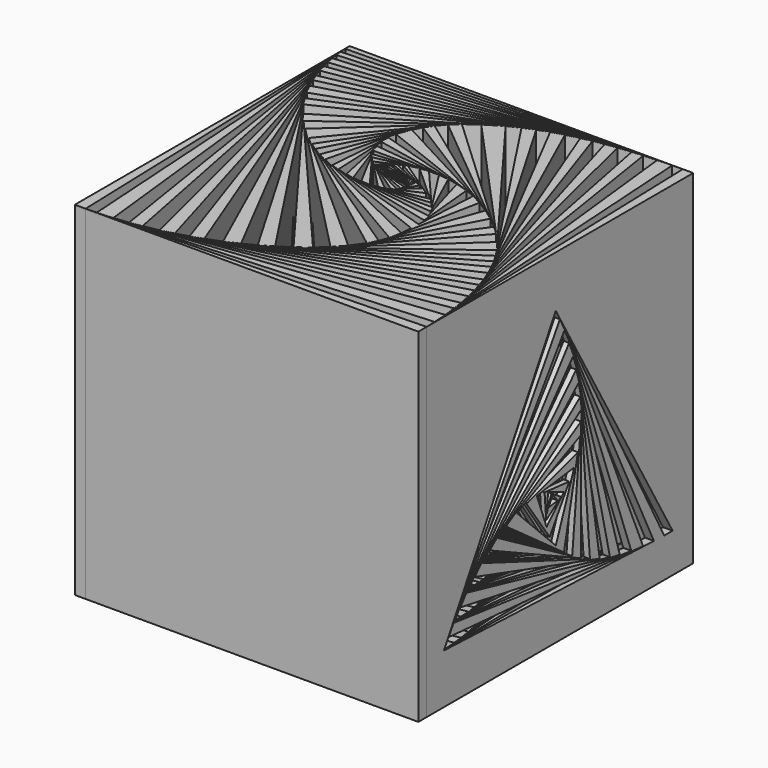
from build123d import *

# Parameters (mm, degrees)
F1_DEPTH = 254
F3_DEPTH = 254.001


with BuildPart() as f1:
    # F0 (on Top) → F1 (new body)
    with BuildSketch(Plane.XY):
        Polygon((-126.8681881938, 122.7877680736), (-127, 127), (-127, -127), (-119.0516725183, -127), align=None)
        Polygon((119.2926133431, 127), (-127, 127), (-126.8681881938, 122.7877680736), (111.5874118838, 126.8681508372), align=None)
    extrude(amount=F1_DEPTH)


with BuildPart() as f1b:
    # F0 (on Top) → F1, piece 2 (new body)
    with BuildSketch(Plane.XY):
        Polygon((-126.0531846551, 113.5256776399), (-126.5785198377, 118.234531984), (-110.9932006372, -126.7478292381), (-99.3302639061, -126.005855037), align=None)
        Polygon((100.7129844798, 126.4739481031), (-126.5785198377, 118.234531984), (-126.0531846551, 113.5256776399), (90.920474554, 125.9147991458), align=None)
    extrude(amount=F1_DEPTH)


with BuildPart() as f1c:
    # F0 (on Top) → F1, piece 3 (new body)
    with BuildSketch(Plane.XY):
        Polygon((-125.3309426111, 108.9235324963), (-88.6490839555, -124.8142276878), (-79.7889641882, -123.4237563291), (-124.2173594964, 103.2422242495), align=None)
        Polygon((82.861461887, 125.281587882), (-125.3309426111, 108.9235324963), (-124.2173594964, 103.2422242495), (73.0560890227, 124.2380037209), align=None)
    extrude(amount=F1_DEPTH)


with BuildPart() as f1d:
    # F0 (on Top) → F1, piece 4 (new body)
    with BuildSketch(Plane.XY):
        Polygon((-122.9498802149, 98.0990388663), (-68.8848311302, -121.2864566216), (-59.508664245, -118.9758074069), (-121.2575487035, 92.3084404823), align=None)
        Polygon((64.6451510187, 123.1163378158), (-122.9498802149, 98.0990388663), (-121.2575487035, 92.3084404823), (56.6793703964, 121.7962442832), align=None)
    extrude(amount=F1_DEPTH)


with BuildPart() as f1e:
    # F0 (on Top) → F1, piece 5 (new body)
    with BuildSketch(Plane.XY):
        Polygon((-119.2080548208, 86.2513609913), (-50.643371318, -116.3848809459), (-42.072519088, -113.4848184256), (-116.9805984588, 80.4835443898), align=None)
        Polygon((48.9444702898, 120.2331074005), (-119.2080548208, 86.2513609913), (-116.9805984588, 80.4835443898), (39.418420978, 117.9510152476), align=None)
    extrude(amount=F1_DEPTH)


with BuildPart() as f1f:
    # F0 (on Top) → F1, piece 6 (new body)
    with BuildSketch(Plane.XY):
        Polygon((-114.0299334632, 73.9299803487), (-31.4888725769, -109.3975506806), (-21.7236330528, -105.0008666387), (-110.0116567717, 66.1407650009), align=None)
        Polygon((30.5370410153, 115.4031382194), (-114.0299334632, 73.9299803487), (-110.0116567717, 66.1407650009), (22.4576933662, 112.5713237272), align=None)
    extrude(amount=F1_DEPTH)


with BuildPart() as f1g:
    # F0 (on Top) → F1, piece 7 (new body)
    with BuildSketch(Plane.XY):
        Polygon((-106.4882692452, 60.0895785941), (-12.9864915382, -100.4935766831), (-4.2246983161, -95.3919006028), (-102.1543719548, 53.5003234443), align=None)
        Polygon((14.2621881215, 109.2357061648), (-106.4882692452, 60.0895785941), (-102.1543719548, 53.5003234443), (5.7810312128, 105.1752827516), align=None)
    extrude(amount=F1_DEPTH)


with BuildPart() as f1h:
    # F0 (on Top) → F1, piece 8 (new body)
    with BuildSketch(Plane.XY):
        Polygon((-95.2082875467, 44.2061987353), (4.7235736363, -89.5064263442), (13.7388739494, -82.7687249575), (-89.3516796687, 37.3804831481), align=None)
        Polygon((-6.3725892117, 97.8379215944), (-95.2082875467, 44.2061987353), (-89.3516796687, 37.3804831481), (-15.4159002419, 91.2490879865), align=None)
    extrude(amount=F1_DEPTH)


with BuildPart() as f1i:
    # F0 (on Top) → F1, piece 9 (new body)
    with BuildSketch(Plane.XY):
        Polygon((-82.4406216858, 30.2987939235), (21.2429796219, -75.9447137933), (28.1362773895, -68.2066711256), (-73.7012457184, 22.5134761845), align=None)
        Polygon((-21.4167941901, 85.7920529864), (-82.4406216858, 30.2987939235), (-73.7012457184, 22.5134761845), (-26.4319034603, 79.7223904415), align=None)
    extrude(amount=F1_DEPTH)


with BuildPart() as f1j:
    # F0 (on Top) → F1, piece 10 (new body)
    with BuildSketch(Plane.XY):
        Polygon((-67.6123478435, 17.92552461), (34.6745146372, -59.1470723376), (38.187583362, -52.5778597304), (-62.191322811, 14.3130401118), align=None)
        Polygon((-30.3811760363, 73.7959690255), (-67.6123478435, 17.92552461), (-62.191322811, 14.3130401118), (-33.6265531217, 67.7273225702), align=None)
    extrude(amount=F1_DEPTH)


with BuildPart() as f1k:
    # F0 (on Top) → F1, piece 11 (new body)
    with BuildSketch(Plane.XY):
        Polygon((-55.9045816766, 10.6394204058), (40.63624374, -45.7736354381), (42.3923361661, -36.9523441909), (-49.5893935967, 7.5818378175), align=None)
        Polygon((-37.5137914336, 57.7661951799), (-55.9045816766, 10.6394204058), (-49.5893935967, 7.5818378175), align=None)
    extrude(amount=F1_DEPTH)


with BuildPart() as f1l:
    # F0 (on Top) → F1, piece 12 (new body)
    with BuildSketch(Plane.XY):
        Polygon((-41.9461483319, 4.5991316782), (42.8538182602, -28.4932750414), (43.2045911016, -22.0635310509), (-35.8799262071, 2.699657456), align=None)
        Polygon((42.3923361661, -36.9523441909), (53.9119721681, 20.913667144), (45.7862644887, 25.2591147985), (43.2045911016, -22.0635310509), (42.8538182602, -28.4932750414), align=None)
        Polygon((29.1134557679, 30.991217705), (-38.0250574646, 51.6334504213), (-37.7312351463, 44.9309046261), (21.4549733149, 32.5883056147), align=None)
        Polygon((-37.7312351463, 44.9309046261), (-38.0250574646, 51.6334504213), (-41.9461483319, 4.5991316782), (-35.8799262071, 2.699657456), align=None)
    extrude(amount=F1_DEPTH)


with BuildPart() as f1m:
    # F0 (on Top) → F1, piece 13 (new body)
    with BuildSketch(Plane.XY):
        Polygon((-28.5686212395, 0.9403759842), (42.6506705396, -16.196753573), (40.9614547645, -10.3084917096), (-22.7560883308, 0), align=None)
        Polygon((42.6506705396, -16.196753573), (38.4668684028, 28.1154417754), (29.1134557679, 30.991217705), (40.9614547645, -10.3084917096), align=None)
        Polygon((13.8678958486, 33.4607075332), (-36.5496441153, 39.2579804339), (-34.5127332434, 33.4607075332), (6.4919767901, 33.4607075332), align=None)
        Polygon((-36.5496441153, 39.2579804339), (-28.5686212395, 0.9403759842), (-22.7560883308, 0), (-34.5127332434, 33.4607075332), align=None)
    extrude(amount=F1_DEPTH)


with BuildPart() as f1n:
    # F0 (on Top) → F1, piece 14 (new body)
    with BuildSketch(Plane.XY):
        Polygon((-16.3723659513, -0.53218918), (38.5998311843, -5.1150339177), (35.6616473557, -0.53218918), (-10.06167382, -0.53218918), align=None)
        Polygon((38.5998311843, -5.1150339177), (21.4549733149, 32.5883056147), (13.8678958486, 33.4607075332), (35.6616473557, -0.53218918), align=None)
        Polygon((0, 32.847757844), (-32.5457947044, 29.7748980058), (-30.1643975353, 26.5649343163), (-7.5473354002, 31.2757530868), align=None)
        Polygon((-32.5457947044, 29.7748980058), (-16.3723659513, -0.53218918), (-10.06167382, -0.53218918), (-30.1643975353, 26.5649343163), align=None)
    extrude(amount=F1_DEPTH)


with BuildPart() as f1o:
    # F0 (on Top) → F1, piece 15 (new body)
    with BuildSketch(Plane.XY):
        Polygon((-4.4250614438, 0), (32.2347954518, 3.4612951674), (28.5073621781, 6.8593647764), (0, 0.9216786153), align=None)
        Polygon((32.2347954518, 3.4612951674), (6.4919767901, 33.4607075332), (0, 32.847757844), (28.5073621781, 6.8593647764), align=None)
        Polygon((-10.146825692, 30.0936856058), (-26.41552278, 22.6958130896), (-23.6386533221, 20.4068586177), (-12.6147075733, 28.3218022504), align=None)
        Polygon((-26.41552278, 22.6958130896), (-4.4250614438, 0), (0, 0.9216786153), (-23.6386533221, 20.4068586177), align=None)
    extrude(amount=F1_DEPTH)


with BuildPart() as f1p:
    # F0 (on Top) → F1, piece 16 (new body)
    with BuildSketch(Plane.XY):
        Polygon((3.329507322, 2.4357070944), (22.300748578, 11.0625088306), (17.0034638905, 14.1694764109), (5.6537325265, 4.4301497601), align=None)
        Polygon((22.300748578, 11.0625088306), (-7.5473354002, 31.2757530868), (-10.146825692, 30.0936856058), (17.0034638905, 14.1694764109), align=None)
        Polygon((-14.1419558573, 26.6465228342), (-21.2695208096, 18.8281065506), (-19.3345417112, 17.7933227858), (-15.1082700185, 24.9989867473), align=None)
        Polygon((-21.2695208096, 18.8281065506), (3.329507322, 2.4357070944), (5.6537325265, 4.4301497601), (-19.3345417112, 17.7933227858), align=None)
    extrude(amount=F1_DEPTH)


with BuildPart() as f1q:
    # F0 (on Top) → F1, piece 17 (new body)
    with BuildSketch(Plane.XY):
        Polygon((7.0708972275, 6.5567984207), (13.3175243975, 15.9307133189), (9.3487022791, 17.4795096335), (7.6296184466, 9.2360226677), align=None)
        Polygon((13.3175243975, 15.9307133189), (-12.6147075733, 28.3218022504), (-14.1419558573, 26.6465228342), (9.3487022791, 17.4795096335), align=None)
        Polygon((-15.6042921852, 22.9375944176), (-17.0736371197, 16.8312213949), (-14.9665841049, 16.1833923534), (-15.3697161374, 20.4531127634), align=None)
        Polygon((-17.0736371197, 16.8312213949), (7.0708972275, 6.5567984207), (7.6296184466, 9.2360226677), (-14.9665841049, 16.1833923534), align=None)
    extrude(amount=F1_DEPTH)


with BuildPart() as f1r:
    # F0 (on Top) → F1, piece 18 (new body)
    with BuildSketch(Plane.XY):
        Polygon((7.4143406474, 11.5161094355), (6.7766325671, 18.2703114997), (4.0880434359, 18.8309856571), (6.4859856679, 13.5576593431), align=None)
        Polygon((6.7766325671, 18.2703114997), (-15.1082700185, 24.9989867473), (-15.6042921852, 22.9375944176), (4.0880434359, 18.8309856571), align=None)
        Polygon((-13.2669719556, 15.8289579035), (7.4143406474, 11.5161094355), (6.4859856679, 13.5576593431), (-10.9204565094, 15.5591432633), align=None)
    extrude(amount=F1_DEPTH)


with BuildPart() as f1s:
    # F0 (on Top) → F1, piece 19 (new body)
    with BuildSketch(Plane.XY):
        Polygon((5.5390247102, 14.6612009808), (1.7969907997, 19.0219829078), (0.2486957437, 19.0219829078), (4.4496764816, 15.5591432633), align=None)
        Polygon((1.7969907997, 19.0219829078), (-15.3697161374, 20.4531127634), (-14.7189377641, 19.0219829078), (0.2486957437, 19.0219829078), align=None)
        Polygon((-12.6174739078, 17.1062087167), (-10.9204565094, 15.5591432633), (-10.064965114, 15.5591432633), (-11.738615487, 16.5735361145), align=None)
        Polygon((-10.064965114, 15.5591432633), (-10.9204565094, 15.5591432633), (5.5390247102, 14.6612009808), (4.4496764816, 15.5591432633), align=None)
    extrude(amount=F1_DEPTH)


with BuildPart() as f1t:
    # F0 (on Top) → F1, piece 20 (new body)
    with BuildSketch(Plane.XY):
        Polygon((3.1098938176, 16.3492539877), (-1.1916278715, 18.8859926014), (-2.9219602182, 18.6164617837), (1.7273046558, 16.8689311728), align=None)
        Polygon((-1.1916278715, 18.8859926014), (-13.3142508724, 17.7414170367), (-12.6174739078, 17.1062087167), (-2.9219602182, 18.6164617837), align=None)
        Polygon((-8.9286324178, 15.652896964), (-9.4015419048, 15.59892948), (3.1098938176, 16.3492539877), (1.7273046558, 16.8689311728), align=None)
    extrude(amount=F1_DEPTH)


with BuildPart() as f1u:
    # F0 (on Top) → F1, piece 21 (new body)
    with BuildSketch(Plane.XY):
        Polygon((0, 17.313343478), (-4.0494421258, 18.355210588), (-4.7813779261, 18.1290722784), (-1.1912890983, 17.5165838079), align=None)
        Polygon((-4.0494421258, 18.355210588), (-11.738615487, 16.5735361145), (-10.9204565094, 16.2323473844), (-4.7813779261, 18.1290722784), align=None)
    extrude(amount=F1_DEPTH)


with BuildPart() as f1v:
    # F0 (on Top) → F1, piece 22 (new body)
    with BuildSketch(Plane.XY):
        Polygon((-110.9932006372, -126.7478292381), (-119.0516725183, -127), (127, -127), (127, -119.3003965724), align=None)
    extrude(amount=F1_DEPTH)


with BuildPart() as f1w:
    # F0 (on Top) → F1, piece 23 (new body)
    with BuildSketch(Plane.XY):
        Polygon((-99.3302639061, -126.005855037), (126.7597363266, -111.6224324751), (126.0749811203, -100.8589091133), (-88.6490839555, -124.8142276878), align=None)
    extrude(amount=F1_DEPTH)


with BuildPart() as f1x:
    # F0 (on Top) → F1, piece 24 (new body)
    with BuildSketch(Plane.XY):
        Polygon((-79.7889641882, -123.4237563291), (125.0067665699, -91.2839427063), (123.7884670629, -83.5209064689), (-68.8848311302, -121.2864566216), align=None)
    extrude(amount=F1_DEPTH)


with BuildPart() as f1y:
    # F0 (on Top) → F1, piece 25 (new body)
    with BuildSketch(Plane.XY):
        Polygon((-59.508664245, -118.9758074069), (121.971694282, -74.2520462948), (120.0602759953, -66.4958811748), (-50.643371318, -116.3848809459), align=None)
    extrude(amount=F1_DEPTH)


with BuildPart() as f1z:
    # F0 (on Top) → F1, piece 26 (new body)
    with BuildSketch(Plane.XY):
        Polygon((-42.072519088, -113.4848184256), (117.9669793997, -59.3333129651), (115.6765473087, -52.5641640735), (-31.4888725769, -109.3975506806), align=None)
    extrude(amount=F1_DEPTH)


with BuildPart() as f1ba:
    # F0 (on Top) → F1, piece 27 (new body)
    with BuildSketch(Plane.XY):
        Polygon((-21.7236330528, -105.0008666387), (112.5755030706, -44.5342629076), (109.3546509415, -37.3806006902), (-12.9864915382, -100.4935766831), align=None)
    extrude(amount=F1_DEPTH)


with BuildPart() as f1bb:
    # F0 (on Top) → F1, piece 28 (new body)
    with BuildSketch(Plane.XY):
        Polygon((-4.2246983161, -95.3919006028), (106.1326003079, -31.1348271478), (102.6265838163, -25.1134743513), (4.7235736363, -89.5064263442), align=None)
    extrude(amount=F1_DEPTH)


with BuildPart() as f1bc:
    # F0 (on Top) → F1, piece 29 (new body)
    with BuildSketch(Plane.XY):
        Polygon((13.7388739494, -82.7687249575), (98.7566325819, -19.2296025397), (92.6280150254, -11.0292795206), (21.2429796219, -75.9447137933), align=None)
    extrude(amount=F1_DEPTH)


with BuildPart() as f1bd:
    # F0 (on Top) → F1, piece 30 (new body)
    with BuildSketch(Plane.XY):
        Polygon((28.1362773895, -68.2066711256), (85.7800778228, -3.4988632934), (79.2486770731, 2.6163682787), (34.6745146372, -59.1470723376), align=None)
    extrude(amount=F1_DEPTH)


with BuildPart() as f1be:
    # F0 (on Top) → F1, piece 31 (new body)
    with BuildSketch(Plane.XY):
        Polygon((38.187583362, -52.5778597304), (71.2420660685, 9.2318973586), (62.6601550053, 15.4253913403), (40.63624374, -45.7736354381), align=None)
    extrude(amount=F1_DEPTH)


with BuildPart() as f1bf:
    # F0 (on Top) → F1, piece 32 (new body)
    with BuildSketch(Plane.XY):
        Polygon((-5.6499548223, 17.7598250391), (-9.9245444636, 15.9426221742), (-8.2313078699, 15.782577531), (-1.1912890983, 17.5165838079), align=None)
    extrude(amount=F1_DEPTH)


with BuildPart() as f1bg:
    # F0 (on Top) → F1, piece 33 (new body)
    with BuildSketch(Plane.XY):
        Polygon((127, 127), (119.2926133431, 127), (126.7597363266, -111.6224324751), (127, -119.3003965724), align=None)
    extrude(amount=F1_DEPTH)


with BuildPart() as f1bh:
    # F0 (on Top) → F1, piece 34 (new body)
    with BuildSketch(Plane.XY):
        Polygon((126.0749811203, -100.8589091133), (111.5874118838, 126.8681508372), (100.7129844798, 126.4739481031), (125.0067665699, -91.2839427063), align=None)
    extrude(amount=F1_DEPTH)


with BuildPart() as f1bi:
    # F0 (on Top) → F1, piece 35 (new body)
    with BuildSketch(Plane.XY):
        Polygon((123.7884670629, -83.5209064689), (90.920474554, 125.9147991458), (82.861461887, 125.281587882), (121.971694282, -74.2520462948), align=None)
    extrude(amount=F1_DEPTH)


with BuildPart() as f1bj:
    # F0 (on Top) → F1, piece 36 (new body)
    with BuildSketch(Plane.XY):
        Polygon((120.0602759953, -66.4958811748), (73.0560890227, 124.2380037209), (64.6451510187, 123.1163378158), (117.9669793997, -59.3333129651), align=None)
    extrude(amount=F1_DEPTH)


with BuildPart() as f1bk:
    # F0 (on Top) → F1, piece 37 (new body)
    with BuildSketch(Plane.XY):
        Polygon((115.6765473087, -52.5641640735), (56.6793703964, 121.7962442832), (48.9444702898, 120.2331074005), (112.5755030706, -44.5342629076), align=None)
    extrude(amount=F1_DEPTH)


with BuildPart() as f1bl:
    # F0 (on Top) → F1, piece 38 (new body)
    with BuildSketch(Plane.XY):
        Polygon((109.3546509415, -37.3806006902), (39.418420978, 117.9510152476), (30.5370410153, 115.4031382194), (106.1326003079, -31.1348271478), align=None)
    extrude(amount=F1_DEPTH)


with BuildPart() as f1bm:
    # F0 (on Top) → F1, piece 39 (new body)
    with BuildSketch(Plane.XY):
        Polygon((102.6265838163, -25.1134743513), (22.4576933662, 112.5713237272), (14.2621881215, 109.2357061648), (98.7566325819, -19.2296025397), align=None)
    extrude(amount=F1_DEPTH)


with BuildPart() as f1bn:
    # F0 (on Top) → F1, piece 40 (new body)
    with BuildSketch(Plane.XY):
        Polygon((92.6280150254, -11.0292795206), (5.7810312128, 105.1752827516), (-6.3725892117, 97.8379215944), (85.7800778228, -3.4988632934), align=None)
    extrude(amount=F1_DEPTH)


with BuildPart() as f1bo:
    # F0 (on Top) → F1, piece 41 (new body)
    with BuildSketch(Plane.XY):
        Polygon((79.2486770731, 2.6163682787), (-15.4159002419, 91.2490879865), (-21.4167941901, 85.7920529864), (71.2420660685, 9.2318973586), align=None)
    extrude(amount=F1_DEPTH)


with BuildPart() as f1bp:
    # F0 (on Top) → F1, piece 42 (new body)
    with BuildSketch(Plane.XY):
        Polygon((62.6601550053, 15.4253913403), (-26.4319034603, 79.7223904415), (-30.3811760363, 73.7959690255), (53.9119721681, 20.913667144), align=None)
    extrude(amount=F1_DEPTH)


with BuildPart() as f1bq:
    # F0 (on Top) → F1, piece 43 (new body)
    with BuildSketch(Plane.XY):
        Polygon((45.7862644887, 25.2591147985), (-33.6265531217, 67.7273225702), (-37.5137914336, 57.7661951799), (38.4668684028, 28.1154417754), align=None)
    extrude(amount=F1_DEPTH)


with BuildPart() as f3_tool:
    # F2 (on face) → F3 (new body, through all)
    with BuildSketch(Plane(origin=(-127, 0, 0), x_dir=(0, -1, 0), z_dir=(-1, 0, 0))):
        Polygon((103.3771738102, 36.8454826179), (0, 215.9), (-3.7791555517, 208.8486365594), (99.0717909055, 43.7563150712), align=None)
        Polygon((94.0431740259, 51.0921703664), (-8.0494379153, 200.0270854402), (-12.3357740902, 189.99055147), (88.2223074085, 58.6924424511), align=None)
        Polygon((82.0971959311, 65.8135734606), (-16.0021610074, 179.8651095474), (-18.9034574402, 169.9911055643), (74.9659300169, 73.169146508), align=None)
        Polygon((68.1151521305, 79.3972333997), (-21.0984706764, 160.5019201916), (-22.6333707181, 150.8463855724), (61.1822067235, 84.8557582973), align=None)
        Polygon((53.6994701863, 89.9077564766), (-23.36179232, 141.9359624606), (-23.36179232, 134.3990971287), (46.0273485724, 94.3372579557), align=None)
        Polygon((35.9812817443, 98.869913505), (-22.4685998115, 125.2417448417), (-20.4050443289, 115.6127381208), (27.1646843847, 101.4878308899), align=None)
        Polygon((17.5494073568, 102.7005953134), (-17.0823343388, 107.0686591901), (-12.4834389782, 99.7712427545), (10.3857171375, 102.0018611994), align=None)
        Polygon((7.14341689, 100.7409618666), (-7.7105512171, 94.9643967597), (-4.852518335, 92.9396856804), (3.9850833442, 98.6870134402), align=None)
        Polygon((3.0305174599, 97.5492240061), (-1.9085433695, 91.6621382446), (6.5184300765, 90.6902700663), align=None)
        Polygon((0, 215.9), (-107.95, 28.9251153229), (-100.2085879445, 28.9251153229), (-3.7791555517, 208.8486365594), align=None)
        Polygon((-8.0494379153, 200.0270854402), (-90.6962892295, 29.2951849142), (-80.6371084746, 30.0617370239), (-12.3357740902, 189.99055147), align=None)
        Polygon((-16.0021610074, 179.8651095474), (-69.7717697899, 31.36985708), (-59.092118036, 33.2167345197), (-18.9034574402, 169.9911055643), align=None)
        Polygon((-21.0984706764, 160.5019201916), (-50.0593477747, 35.3021597486), (-40.5427616907, 38.1844923904), (-22.6333707181, 150.8463855724), align=None)
        Polygon((-23.36179232, 141.9359624606), (-31.5650422395, 41.5896417586), (-23.36179232, 45.4164158245), (-23.36179232, 134.3990971287), align=None)
        Polygon((-22.4685998115, 125.2417448417), (-15.1452764007, 50.1602235023), (-7.5531639995, 55.6430192997), (-20.4050443289, 115.6127381208), align=None)
        Polygon((-17.0823343388, 107.0686591901), (0, 63.1428235477), (5.609748658, 71.0614082231), (-12.4834389782, 99.7712427545), align=None)
        Polygon((-7.7105512171, 94.9643967597), (8.4776201534, 78.6610494761), (8.8512554258, 83.2315459539), (-4.852518335, 92.9396856804), align=None)
        Polygon((8.4681653884, 87.1591319961), (7.14341689, 100.7409618666), (3.9850833442, 98.6870134402), align=None)
        Polygon((8.4776201534, 78.6610494761), (17.5494073568, 102.7005953134), (10.3857171375, 102.0018611994), (8.8512554258, 83.2315459539), align=None)
        Polygon((0, 63.1428235477), (35.9812817443, 98.869913505), (27.1646843847, 101.4878308899), (5.609748658, 71.0614082231), align=None)
        Polygon((-15.1452764007, 50.1602235023), (53.6994701863, 89.9077564766), (46.0273485724, 94.3372579557), (-7.5531639995, 55.6430192997), align=None)
        Polygon((-31.5650422395, 41.5896417586), (68.1151521305, 79.3972333997), (61.1822067235, 84.8557582973), (-23.36179232, 45.4164158245), align=None)
        Polygon((-50.0593477747, 35.3021597486), (82.0971959311, 65.8135734606), (74.9659300169, 73.169146508), (-40.5427616907, 38.1844923904), align=None)
        Polygon((-69.7717697899, 31.36985708), (94.0431740259, 51.0921703664), (88.2223074085, 58.6924424511), (-59.092118036, 33.2167345197), align=None)
        Polygon((-80.6371084746, 30.0617370239), (-90.6962892295, 29.2951849142), (103.3771738102, 36.8454826179), (99.0717909055, 43.7563150712), align=None)
    extrude(amount=-F3_DEPTH)


with BuildPart() as f1_1:
    add(f1.part)

    # F3: cut by f3_tool
    add(f3_tool.part, mode=Mode.SUBTRACT)


with BuildPart() as f1b_1:
    add(f1b.part)

    # F3: cut by f3_tool
    add(f3_tool.part, mode=Mode.SUBTRACT)


with BuildPart() as f1c_1:
    add(f1c.part)

    # F3: cut by f3_tool
    add(f3_tool.part, mode=Mode.SUBTRACT)


with BuildPart() as f1d_1:
    add(f1d.part)

    # F3: cut by f3_tool
    add(f3_tool.part, mode=Mode.SUBTRACT)


with BuildPart() as f1e_1:
    add(f1e.part)

    # F3: cut by f3_tool
    add(f3_tool.part, mode=Mode.SUBTRACT)


with BuildPart() as f1f_1:
    add(f1f.part)

    # F3: cut by f3_tool
    add(f3_tool.part, mode=Mode.SUBTRACT)


with BuildPart() as f1g_1:
    add(f1g.part)

    # F3: cut by f3_tool
    add(f3_tool.part, mode=Mode.SUBTRACT)


with BuildPart() as f1h_1:
    add(f1h.part)

    # F3: cut by f3_tool
    add(f3_tool.part, mode=Mode.SUBTRACT)


with BuildPart() as f1i_1:
    add(f1i.part)

    # F3: cut by f3_tool
    add(f3_tool.part, mode=Mode.SUBTRACT)


with BuildPart() as f1j_1:
    add(f1j.part)

    # F3: cut by f3_tool
    add(f3_tool.part, mode=Mode.SUBTRACT)


with BuildPart() as f1k_1:
    add(f1k.part)

    # F3: cut by f3_tool
    add(f3_tool.part, mode=Mode.SUBTRACT)


with BuildPart() as f1l_1:
    add(f1l.part)

    # F3: cut by f3_tool
    add(f3_tool.part, mode=Mode.SUBTRACT)


with BuildPart() as f1m_1:
    add(f1m.part)

    # F3: cut by f3_tool
    add(f3_tool.part, mode=Mode.SUBTRACT)


with BuildPart() as f1n_1:
    add(f1n.part)

    # F3: cut by f3_tool
    add(f3_tool.part, mode=Mode.SUBTRACT)


with BuildPart() as f1o_1:
    add(f1o.part)

    # F3: cut by f3_tool
    add(f3_tool.part, mode=Mode.SUBTRACT)


with BuildPart() as f1p_1:
    add(f1p.part)

    # F3: cut by f3_tool
    add(f3_tool.part, mode=Mode.SUBTRACT)


with BuildPart() as f1q_1:
    add(f1q.part)

    # F3: cut by f3_tool
    add(f3_tool.part, mode=Mode.SUBTRACT)


with BuildPart() as f1r_1:
    add(f1r.part)

    # F3: cut by f3_tool
    add(f3_tool.part, mode=Mode.SUBTRACT)


with BuildPart() as f1s_1:
    add(f1s.part)

    # F3: cut by f3_tool
    add(f3_tool.part, mode=Mode.SUBTRACT)


with BuildPart() as f1t_1:
    add(f1t.part)

    # F3: cut by f3_tool
    add(f3_tool.part, mode=Mode.SUBTRACT)


with BuildPart() as f1u_1:
    add(f1u.part)

    # F3: cut by f3_tool
    add(f3_tool.part, mode=Mode.SUBTRACT)


with BuildPart() as f1w_1:
    add(f1w.part)

    # F3: cut by f3_tool
    add(f3_tool.part, mode=Mode.SUBTRACT)


with BuildPart() as f1x_1:
    add(f1x.part)

    # F3: cut by f3_tool
    add(f3_tool.part, mode=Mode.SUBTRACT)


with BuildPart() as f1y_1:
    add(f1y.part)

    # F3: cut by f3_tool
    add(f3_tool.part, mode=Mode.SUBTRACT)


with BuildPart() as f1z_1:
    add(f1z.part)

    # F3: cut by f3_tool
    add(f3_tool.part, mode=Mode.SUBTRACT)


with BuildPart() as f1ba_1:
    add(f1ba.part)

    # F3: cut by f3_tool
    add(f3_tool.part, mode=Mode.SUBTRACT)


with BuildPart() as f1bb_1:
    add(f1bb.part)

    # F3: cut by f3_tool
    add(f3_tool.part, mode=Mode.SUBTRACT)


with BuildPart() as f1bc_1:
    add(f1bc.part)

    # F3: cut by f3_tool
    add(f3_tool.part, mode=Mode.SUBTRACT)


with BuildPart() as f1bd_1:
    add(f1bd.part)

    # F3: cut by f3_tool
    add(f3_tool.part, mode=Mode.SUBTRACT)


with BuildPart() as f1be_1:
    add(f1be.part)

    # F3: cut by f3_tool
    add(f3_tool.part, mode=Mode.SUBTRACT)


with BuildPart() as f1bf_1:
    add(f1bf.part)

    # F3: cut by f3_tool
    add(f3_tool.part, mode=Mode.SUBTRACT)


with BuildPart() as f1bg_1:
    add(f1bg.part)

    # F3: cut by f3_tool
    add(f3_tool.part, mode=Mode.SUBTRACT)


with BuildPart() as f1bh_1:
    add(f1bh.part)

    # F3: cut by f3_tool
    add(f3_tool.part, mode=Mode.SUBTRACT)


with BuildPart() as f1bi_1:
    add(f1bi.part)

    # F3: cut by f3_tool
    add(f3_tool.part, mode=Mode.SUBTRACT)


with BuildPart() as f1bj_1:
    add(f1bj.part)

    # F3: cut by f3_tool
    add(f3_tool.part, mode=Mode.SUBTRACT)


with BuildPart() as f1bk_1:
    add(f1bk.part)

    # F3: cut by f3_tool
    add(f3_tool.part, mode=Mode.SUBTRACT)


with BuildPart() as f1bl_1:
    add(f1bl.part)

    # F3: cut by f3_tool
    add(f3_tool.part, mode=Mode.SUBTRACT)


with BuildPart() as f1bm_1:
    add(f1bm.part)

    # F3: cut by f3_tool
    add(f3_tool.part, mode=Mode.SUBTRACT)


with BuildPart() as f1bn_1:
    add(f1bn.part)

    # F3: cut by f3_tool
    add(f3_tool.part, mode=Mode.SUBTRACT)


with BuildPart() as f1bo_1:
    add(f1bo.part)

    # F3: cut by f3_tool
    add(f3_tool.part, mode=Mode.SUBTRACT)


with BuildPart() as f1bp_1:
    add(f1bp.part)

    # F3: cut by f3_tool
    add(f3_tool.part, mode=Mode.SUBTRACT)


with BuildPart() as f1bq_1:
    add(f1bq.part)

    # F3: cut by f3_tool
    add(f3_tool.part, mode=Mode.SUBTRACT)


solid = Compound([f1v.part, f1_1.part, f1b_1.part, f1c_1.part, f1d_1.part, f1e_1.part, f1f_1.part, f1g_1.part, f1h_1.part, f1i_1.part, f1j_1.part, f1k_1.part, f1l_1.part, f1m_1.part, f1n_1.part, f1o_1.part, f1p_1.part, f1q_1.part, f1r_1.part, f1s_1.part, f1t_1.part, f1u_1.part, f1w_1.part, f1x_1.part, f1y_1.part, f1z_1.part, f1ba_1.part, f1bb_1.part, f1bc_1.part, f1bd_1.part, f1be_1.part, f1bf_1.part, f1bg_1.part, f1bh_1.part, f1bi_1.part, f1bj_1.part, f1bk_1.part, f1bl_1.part, f1bm_1.part, f1bn_1.part, f1bo_1.part, f1bp_1.part, f1bq_1.part])
